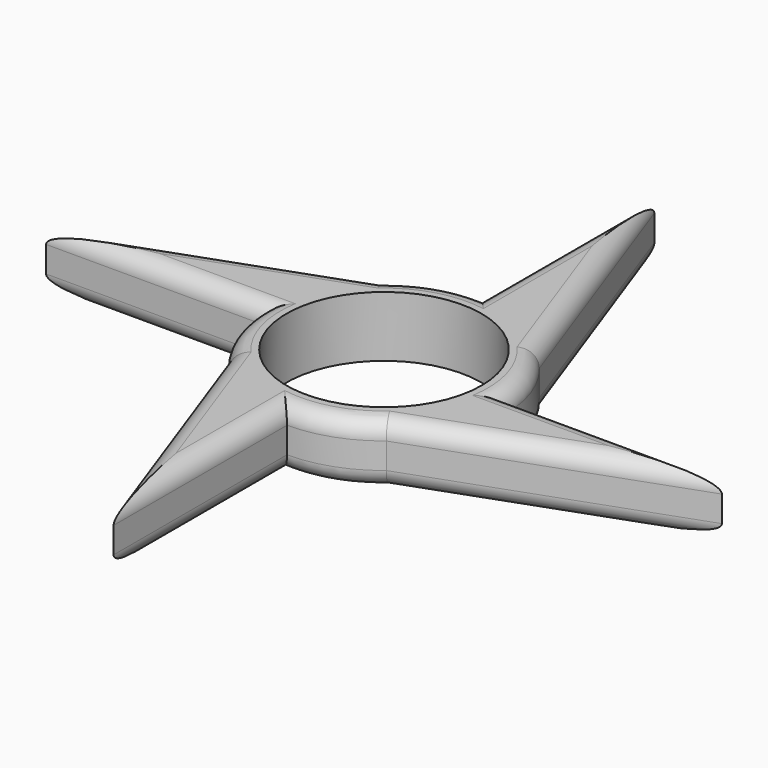
from build123d import *

# Parameters (mm, degrees)
F0_R     = 11.25
F1_DEPTH = 7
F2_R     = 2
F3_R     = 2


with BuildPart() as f1:
    # F0 (on Top) → F1 (new body)
    with BuildSketch(Plane.XY):
        with BuildLine():
            Line((10.8037274316, 8.9039021549), (14, 0))
            ThreePointArc((14, 0), (13.1767253907, 4.7301065505), (10.8037274316, 8.9039021549))
        make_face()
        with BuildLine():
            Line((39, 0), (14, 0))
            ThreePointArc((14, 0), (12.6620422952, -5.97266146), (8.9039021549, -10.8037274316))
            Line((8.9039021549, -10.8037274316), (39, 0))
        make_face()
        with BuildLine():
            ThreePointArc((8.9039021549, -10.8037274316), (12.6620422952, -5.97266146), (14, 0))
            Line((14, 0), (10.8037274316, 8.9039021549))
            ThreePointArc((10.8037274316, 8.9039021549), (5.97266146, 12.6620422952), (0, 14))
            Line((0, 14), (-8.9039021549, 10.8037274316))
            ThreePointArc((-8.9039021549, 10.8037274316), (-12.6620422952, 5.97266146), (-14, 0))
            Line((-14, 0), (-10.8037274316, -8.9039021549))
            ThreePointArc((-10.8037274316, -8.9039021549), (-5.97266146, -12.6620422952), (0, -14))
            Line((0, -14), (8.9039021549, -10.8037274316))
        make_face()
        Circle(F0_R, mode=Mode.SUBTRACT)
        with BuildLine():
            ThreePointArc((0, 14), (5.97266146, 12.6620422952), (10.8037274316, 8.9039021549))
            Line((10.8037274316, 8.9039021549), (0, 39))
            Line((0, 39), (0, 14))
        make_face()
        with BuildLine():
            ThreePointArc((0, -14), (4.7301065505, -13.1767253907), (8.9039021549, -10.8037274316))
            Line((8.9039021549, -10.8037274316), (0, -14))
        make_face()
        with BuildLine():
            Line((-8.9039021549, 10.8037274316), (0, 14))
            ThreePointArc((0, 14), (-4.7301065505, 13.1767253907), (-8.9039021549, 10.8037274316))
        make_face()
        with BuildLine():
            Line((0, -39), (0, -14))
            ThreePointArc((0, -14), (-5.97266146, -12.6620422952), (-10.8037274316, -8.9039021549))
            Line((-10.8037274316, -8.9039021549), (0, -39))
        make_face()
        with BuildLine():
            ThreePointArc((-14, 0), (-12.6620422952, 5.97266146), (-8.9039021549, 10.8037274316))
            Line((-8.9039021549, 10.8037274316), (-39, 0))
            Line((-39, 0), (-14, 0))
        make_face()
        with BuildLine():
            ThreePointArc((-14, 0), (-13.1767253907, -4.7301065505), (-10.8037274316, -8.9039021549))
            Line((-10.8037274316, -8.9039021549), (-14, 0))
        make_face()
    extrude(amount=F1_DEPTH)

    # F2
    f2_edges = [f1.edges().sort_by_distance(p)[0] for p in [
        (0, -26.5, 7),
        (23.951951, -5.401864, 7),
        (5.401864, 23.951951, 7),
        (-23.951951, 5.401864, 7),
        (-26.5, 0, 7),
        (-5.401864, -23.951951, 7),
        (0, 26.5, 7),
        (13.176725, 4.730107, 7),
        (-4.730107, 13.176725, 7),
        (-13.176725, -4.730107, 7),
        (4.730107, -13.176725, 7),
        (26.5, 0, 7),
    ]]
    fillet(f2_edges, radius=F2_R)

    # F3
    f3_edges = [f1.edges().sort_by_distance(p)[0] for p in [
        (-26.5, 0, 0),
        (-5.401864, -23.951951, 0),
        (0, -26.5, 0),
        (23.951951, -5.401864, 0),
        (26.5, 0, 0),
        (5.401864, 23.951951, 0),
        (0, 26.5, 0),
        (-23.951951, 5.401864, 0),
        (4.730107, -13.176725, 0),
        (-13.176725, -4.730107, 0),
        (-4.730107, 13.176725, 0),
        (13.176725, 4.730107, 0),
    ]]
    fillet(f3_edges, radius=F3_R)


solid = f1.part
